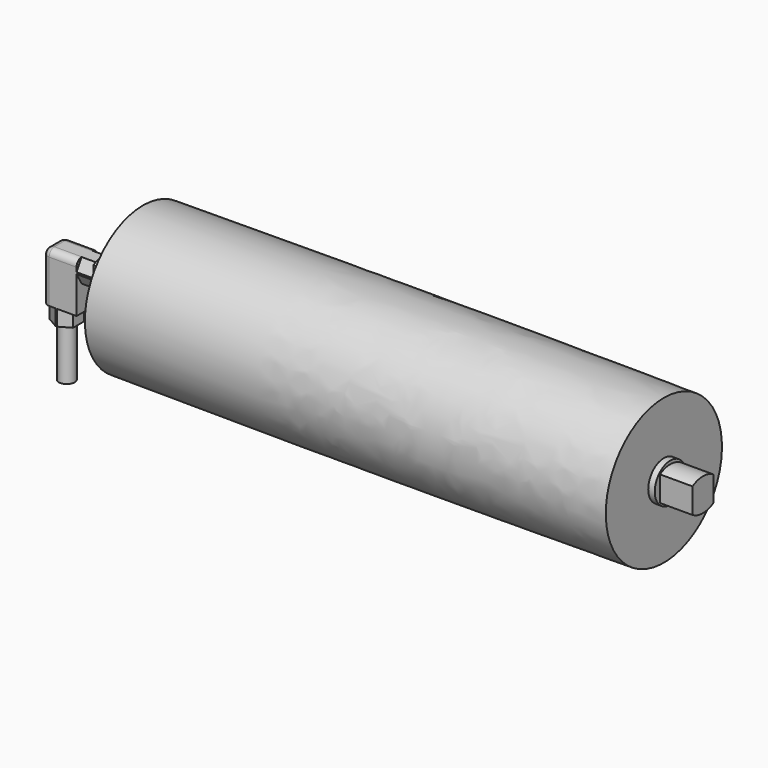
from build123d import *

# Parameters (mm, degrees)
F0_W          = 400
F0_H          = 55.75
F2_W          = 20
F2_H          = 19.3462212823
F3_DEPTH      = 30
F4_R          = 15
F5_DEPTH      = 5
F7_DEPTH      = 13
F9_DEPTH      = 50
F11_DEPTH     = 12
F12_R         = 6
F13_DEPTH     = 40
F14_T1_DEPTH  = 63
F14_T3_DEPTH  = 10
F14_S7_W      = 5.1
F14_S7_H      = 5.1
F14_T8_DEPTH  = 5.1
F14_S13_W     = 5.1
F14_S13_H     = 5.1
F14_T14_DEPTH = 5.1
F14_T20_DEPTH = 51
F14_T25_DEPTH = 51


# Not quite as in the source:
# - a fillet or chamfer that OpenCascade refuses, or shapes differently, is made with other operations: its cross-section is extruded or revolved along the edge and cut away or added
# - a pattern or mirror of a feature is missing from the dataset's text; its kind, count and spacing are read off the source's solid


with BuildPart() as f1:
    # F0 (on Front) → F1 (revolve)
    with BuildSketch(Plane.XZ):
        with Locations((0, 27.875)):
            Rectangle(F0_W, F0_H)
        with BuildLine():
            ThreePointArc((200, 55.75), (0, 56.5), (-200, 55.75))
            Line((-200, 55.75), (200, 55.75))
        make_face()
    revolve(axis=Axis((0, 0, 0), (1, 0, 0)))

    # F2 (on face) → F3 (join)
    with BuildSketch(Plane(origin=(-200, 0, 0), x_dir=(0, -1, 0), z_dir=(-1, 0, 0))):
        Rectangle(F2_W, F2_H)
        with BuildLine():
            ThreePointArc((-10, -9.6731106412), (0, -12.5), (10, -9.6731106412))
            Line((10, -9.6731106412), (-10, -9.6731106412))
        make_face()
        with BuildLine():
            Line((-10, 9.6731106412), (10, 9.6731106412))
            ThreePointArc((10, 9.6731106412), (0, 12.5), (-10, 9.6731106412))
        make_face()
    f3 = extrude(amount=F3_DEPTH)

    # F3_copies: F3 across plane
    add(f3.mirror(Plane(origin=(0, 0, 0), x_dir=(0, 0, 1), z_dir=(1, 0, 0))))

    # F4 (on face) → F5 (join)
    with BuildSketch(Plane(origin=(-200, 0, 0), x_dir=(0, -1, 0), z_dir=(-1, 0, 0))):
        Circle(F4_R)
        with BuildLine():
            Line((10, 9.6731106412), (10, -9.6731106412))
            ThreePointArc((10, -9.6731106412), (0, -12.5), (-10, -9.6731106412))
            Line((-10, -9.6731106412), (-10, 9.6731106412))
            ThreePointArc((-10, 9.6731106412), (0, 12.5), (10, 9.6731106412))
        make_face(mode=Mode.SUBTRACT)
    f5 = extrude(amount=F5_DEPTH)

    # F5_copies: F5 across plane
    add(f5.mirror(Plane(origin=(0, 0, 0), x_dir=(0, 0, 1), z_dir=(1, 0, 0))))

    # F6 (on face) → F7 (join)
    with BuildSketch(Plane(origin=(-230, 0, 0), x_dir=(0, -1, 0), z_dir=(-1, 0, 0))):
        Polygon((10, 0.6794919243), (5.1961524227, 9), (-5.1961524227, 9), (-10, 0.6794919243), (-10, -0.6794919243), (-5.1961524227, -9), (5.1961524227, -9), (10, -0.6794919243), align=None)
    extrude(amount=F7_DEPTH)

    # F8 (on face) → F9 (join)
    with BuildSketch(Plane.XY.offset(9)):
        Polygon((-243, 10), (-269, 10), (-269, -10), (-243, -10), (-243, -5.1961524227), (-243, 5.1961524227), align=None)
    extrude(amount=-F9_DEPTH)

    # F10 (on face) → F11 (cut)
    with BuildSketch(Plane(origin=(0, 0, -41), x_dir=(1, 0, 0), z_dir=(0, 0, -1))):
        Polygon((-269, -10), (-259.1794919243, -10), (-267.5, -5.1961524227), (-267.5, 5.1961524227), (-259.1794919243, 10), (-269, 10), align=None)
        Polygon((-257.8205080757, -10), (-243, -10), (-243, 10), (-257.8205080757, 10), (-249.5, 5.1961524227), (-249.5, -5.1961524227), align=None)
    extrude(amount=-F11_DEPTH, mode=Mode.SUBTRACT)

    # F12 (on face) → F13 (join)
    with BuildSketch(Plane(origin=(0, 0, -41), x_dir=(1, 0, 0), z_dir=(0, 0, -1))):
        with Locations((-258.5, 0)):
            Circle(F12_R)
    extrude(amount=F13_DEPTH)

    # F14: fillet of radius 5 on 5 edges, made by hand

    # F14_s2 → F14_t1 (cut)
    with BuildSketch(Plane.XY.offset(-59)):
        with BuildLine():
            ThreePointArc((-269, -5), (-267.5355339059, -8.5355339059), (-264, -10))
            Line((-264, -10), (-264, -10.1))
            Line((-264, -10.1), (-269.1, -10.1))
            Line((-269.1, -10.1), (-269.1, -5))
            Line((-269.1, -5), (-269, -5))
        make_face()
        with BuildLine():
            ThreePointArc((-264, 10), (-267.5355339059, 8.5355339059), (-269, 5))
            Line((-269, 5), (-269.1, 5))
            Line((-269.1, 5), (-269.1, 10.1))
            Line((-269.1, 10.1), (-264, 10.1))
            Line((-264, 10.1), (-264, 10))
        make_face()
    extrude(amount=F14_T1_DEPTH, mode=Mode.SUBTRACT)

    # F14_s4 → F14_t3 (cut)
    with BuildSketch(Plane.XZ.offset(-5)):
        with BuildLine():
            ThreePointArc((-264, 9), (-267.5355339059, 7.5355339059), (-269, 4))
            Line((-269, 4), (-269.1, 4))
            Line((-269.1, 4), (-269.1, 9.1))
            Line((-269.1, 9.1), (-264, 9.1))
            Line((-264, 9.1), (-264, 9))
        make_face()
    extrude(amount=F14_T3_DEPTH, mode=Mode.SUBTRACT)


with BuildPart() as f14_tool6:
    # F14_s7 → F14_t8 (new body)
    with BuildSketch(Plane.XZ.offset(5)):
        with Locations((-266.55, 6.55)):
            Rectangle(F14_S7_W, F14_S7_H)
    extrude(amount=F14_T8_DEPTH)

    # F14_s9 → F14_t10 (revolve, cut)
    with BuildSketch(Plane(origin=(-264, -5, 4), x_dir=(0.7071067812, 0, -0.7071067812), z_dir=(-0.7071067812, 0, -0.7071067812))):
        with BuildLine():
            ThreePointArc((0, -5), (5, 0), (0, 5))
            Line((0, 5), (0, -5))
        make_face()
    revolve(axis=Axis((-264, -5, 4), (0, -1, 0)), mode=Mode.SUBTRACT)


with BuildPart() as f1_1:
    add(f1.part)

    # F14_t5: cut F14_tool6
    add(f14_tool6.part, mode=Mode.SUBTRACT)


with BuildPart() as f14_tool12:
    # F14_s13 → F14_t14 (new body)
    with BuildSketch(Plane.XZ.offset(-5)):
        with Locations((-266.55, 6.55)):
            Rectangle(F14_S13_W, F14_S13_H)
    extrude(amount=-F14_T14_DEPTH)

    # F14_s15 → F14_t16 (revolve, cut)
    with BuildSketch(Plane(origin=(-264, 5, 4), x_dir=(0.7071067812, 0, -0.7071067812), z_dir=(0.7071067812, 0, 0.7071067812))):
        with BuildLine():
            ThreePointArc((0, -5), (5, 0), (0, 5))
            Line((0, 5), (0, -5))
        make_face()
    revolve(axis=Axis((-264, 5, 4), (0, 1, 0)), mode=Mode.SUBTRACT)


with BuildPart() as f1_2:
    add(f1_1.part)

    # F14_t11: cut F14_tool12
    add(f14_tool12.part, mode=Mode.SUBTRACT)


with BuildPart() as f14_tool18:
    # F14_s19 → F14_t20 (new body)
    with BuildSketch(Plane.YZ.offset(-264)):
        with BuildLine():
            ThreePointArc((-5, 9), (-8.5355339059, 7.5355339059), (-10, 4))
            Line((-10, 4), (-10.1, 4))
            Line((-10.1, 4), (-10.1, 9.1))
            Line((-10.1, 9.1), (-5, 9.1))
            Line((-5, 9.1), (-5, 9))
        make_face()
    extrude(amount=F14_T20_DEPTH)

    split(bisect_by=Plane.YZ.offset(-230), keep=Keep.BOTTOM)


with BuildPart() as f1_3:
    add(f1_2.part)

    # F14_t17: cut F14_tool18
    add(f14_tool18.part, mode=Mode.SUBTRACT)


with BuildPart() as f14_tool23:
    # F14_s24 → F14_t25 (new body)
    with BuildSketch(Plane.YZ.offset(-213)):
        with BuildLine():
            ThreePointArc((10, 4), (8.5355339059, 7.5355339059), (5, 9))
            Line((5, 9), (5, 9.1))
            Line((5, 9.1), (10.1, 9.1))
            Line((10.1, 9.1), (10.1, 4))
            Line((10.1, 4), (10, 4))
        make_face()
    extrude(amount=-F14_T25_DEPTH)

    split(bisect_by=Plane.YZ.offset(-230), keep=Keep.BOTTOM)


with BuildPart() as f1_4:
    add(f1_3.part)

    # F14_t22: cut F14_tool23
    add(f14_tool23.part, mode=Mode.SUBTRACT)


solid = f1_4.part
